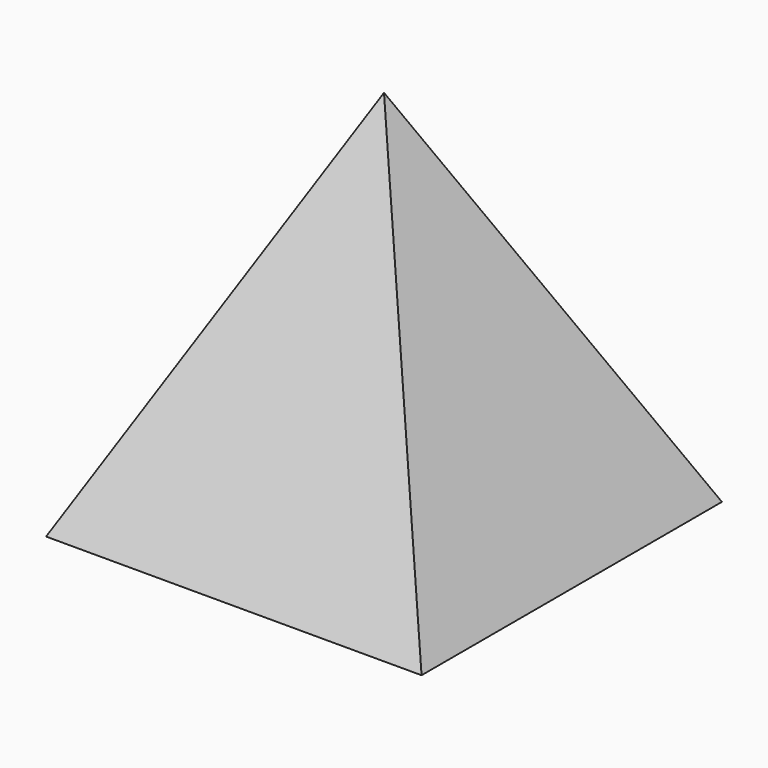
from build123d import *

# Parameters (mm, degrees)
F0_W     = 25.4
F0_H     = 25.4
F1_DEPTH = 25.4
F2_SIZE2 = 25.39999
F2_SIZE  = 12.69999


# Not quite as in the source:
# - a fillet or chamfer is up to 0.001 mm smaller than in the source, because OpenCascade refuses the exact size


with BuildPart() as f1:
    # F0 (on Front) → F1 (new body)
    with BuildSketch(Plane.XZ):
        with Locations((12.7, 12.7)):
            Rectangle(F0_W, F0_H)
    extrude(amount=F1_DEPTH)

    # F2 (size 12.7 and 25.4 in the source; OpenCascade refuses exactly that, so slightly less here)
    f2_edges = [f1.edges().sort_by_distance(p)[0] for p in [
        (25.4, -12.7, 25.4),
        (0, -12.7, 25.4),
        (12.7, 0, 25.4),
        (12.7, -25.4, 25.4),
    ]]
    f2_side = f1.faces().sort_by_distance((12.7, -12.7, 25.4))[0]
    chamfer(f2_edges, length=F2_SIZE, length2=F2_SIZE2, reference=f2_side)


solid = f1.part
